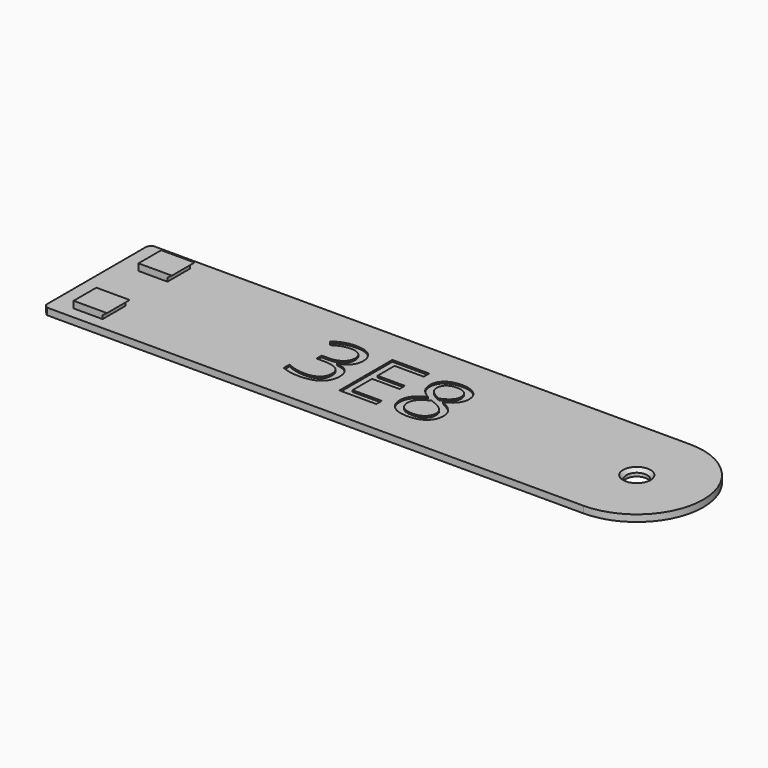
from build123d import *

# Parameters (mm, degrees)
F1_R          = 3.075
F2_DEPTH      = 2
F3_W          = 9.72
F3_H          = 8.4
F4_DEPTH      = 2
F5_SIZE       = 1
F7_DEPTH      = 8.4
F9_DEPTH      = 8.4
F10_TEXT_SIZE = 27.4166666667
F11_DEPTH     = 0.5
F12_W         = 1.15
F12_H         = 8.4
F13_DEPTH     = 2


# Not quite as in the source:
# - Text() gives the source's letters only with a copy of the font that has no kerning and outlines rounded to 1/6400 em; it was checked with that copy


with BuildPart() as f2:
    # F1 (on Top) → F2 (new body)
    with BuildSketch(Plane.XY):
        with BuildLine():
            Line((-84.87, -19.7), (75, -19.7))
            ThreePointArc((75, -19.7), (94.7, 0), (75, 19.7))
            Line((75, 19.7), (-84.87, 19.7))
            Line((-84.87, 19.7), (-84.87, -19.7))
        make_face()
        with Locations((75, 0)):
            Circle(F1_R, mode=Mode.SUBTRACT)
    extrude(amount=F2_DEPTH)

    # F3 (on face) → F4 (join)
    with BuildSketch(Plane.XY.offset(2)):
        with Locations((-75, 12)):
            Rectangle(F3_W, F3_H)
        with Locations((-75, -12)):
            Rectangle(F3_W, F3_H)
    extrude(amount=F4_DEPTH)

    # F5
    f5_edges = [f2.edges().sort_by_distance(p)[0] for p in [
        (71.925, 0, 2),
        (-84.87, -19.7, 1),
        (-84.87, 19.7, 1),
    ]]
    chamfer(f5_edges, length=F5_SIZE)

    # F6 (on face) → F7 (join, through all)
    with BuildSketch(Plane.XZ.offset(16.2)):
        Polygon((-68.84, 4), (-70.14, 4), (-70.14, 3), align=None)
    extrude(amount=-F7_DEPTH)

    # F8 (on face) → F9 (join, through all)
    with BuildSketch(Plane.XZ.offset(-7.8)):
        Polygon((-70.14, 4), (-70.14, 3), (-68.84, 4), align=None)
    extrude(amount=-F9_DEPTH)

    # F10 (on face) → F11 (cut)
    with BuildSketch(Plane.XY.offset(2)):
        with Locations((-23.4776627604, -9.87)):
            Text('3E8', F10_TEXT_SIZE, font='Open Sans', text_align=(TextAlign.LEFT, TextAlign.BOTTOM))
    extrude(amount=-F11_DEPTH, mode=Mode.SUBTRACT)

    # F12 (on face) → F13 (cut, through all)
    with BuildSketch(Plane.XY.offset(4)):
        with Locations((-79.285, 12)):
            Rectangle(F12_W, F12_H)
        with Locations((-79.285, -12)):
            Rectangle(F12_W, F12_H)
    extrude(amount=-F13_DEPTH, mode=Mode.SUBTRACT)


solid = f2.part
